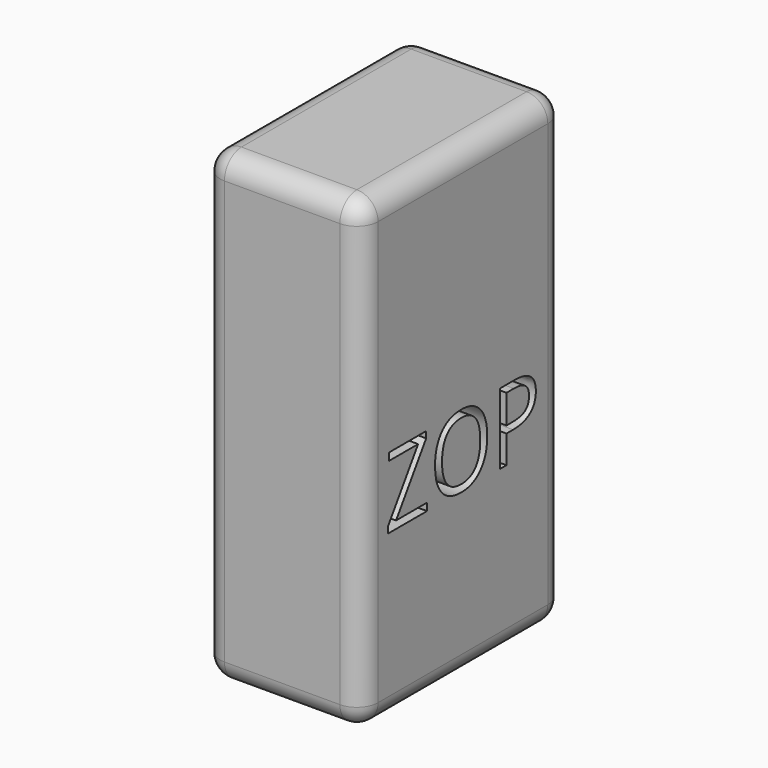
from build123d import *

# Parameters (mm, degrees)
F0_W         = 18.6
F0_H         = 30
F1_DEPTH     = 54.9
F2_R         = 2.5
F3_TEXT_SIZE = 11.7039039517
F4_DEPTH     = 5


# Not quite as in the source:
# - Text() gives the source's letters only with a copy of the font that has no kerning and outlines rounded to 1/6400 em; it was checked with that copy


with BuildPart() as f1:
    # F0 (on Top) → F1 (new body)
    with BuildSketch(Plane.XY):
        Rectangle(F0_W, F0_H)
    extrude(amount=F1_DEPTH)

    # F2
    f2_edges = [f1.edges().sort_by_distance(p)[0] for p in [
        (9.3, 15, 27.45),
        (-9.3, 15, 27.45),
        (0, 15, 0),
        (0, 15, 54.9),
        (0, -15, 54.9),
        (9.3, 0, 54.9),
        (-9.3, 0, 54.9),
        (-9.3, -15, 27.45),
        (9.3, -15, 27.45),
        (0, -15, 0),
        (9.3, 0, 0),
        (-9.3, 0, 0),
    ]]
    fillet(f2_edges, radius=F2_R)

    # F3 (on face) → F4 (cut)
    with BuildSketch(Plane.YZ.offset(9.3)):
        with Locations((-11.5, 19.4400772276)):
            Text('ZOP', F3_TEXT_SIZE, font='Open Sans', text_align=(TextAlign.LEFT, TextAlign.BOTTOM))
    extrude(amount=-F4_DEPTH, mode=Mode.SUBTRACT)


solid = f1.part
